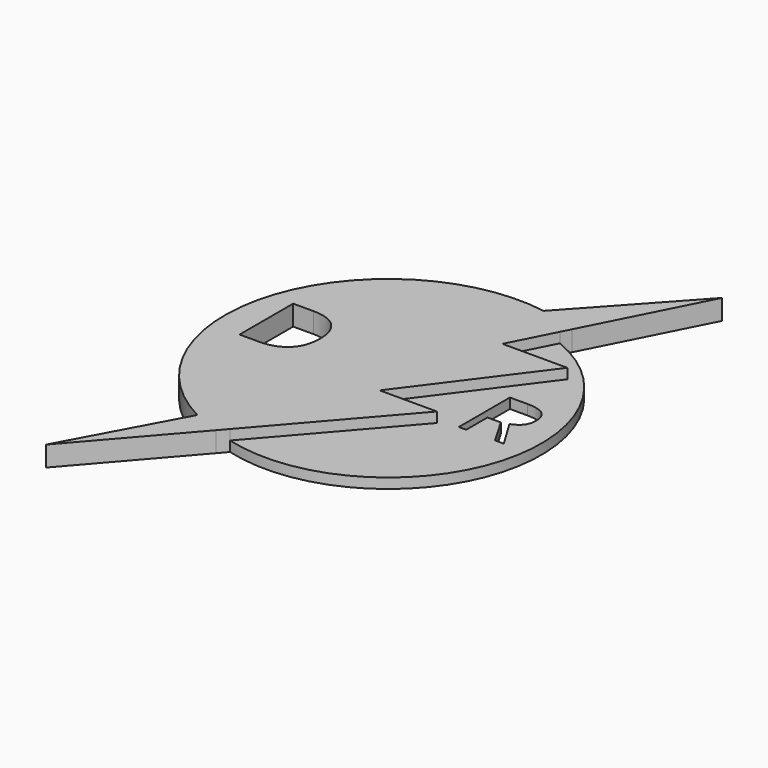
from build123d import *

# Parameters (mm, degrees)
F1_DEPTH = 3.2
F2_DEPTH = 1.6
F3_DEPTH = 2.5


# Not quite as in the source:
# - a feature names something its author has since deleted; it is built from what else it names


with BuildPart() as f1:
    # F0 (on Top) → F1 (new body)
    with BuildSketch(Plane.XY):
        with BuildLine():
            Line((-12.0286401361, 7.7058477327), (2.8731075212, 24.026809333))
            ThreePointArc((2.8731075212, 24.026809333), (-23.1446184854, 7.061795007), (-11.0294978873, -21.5381635686))
            Line((-11.0294978873, -21.5381635686), (-4.3697794008, -9.2094279826))
            Line((-4.3697794008, -9.2094279826), (-18.230907619, -9.2094279826))
            Line((-18.230907619, -9.2094279826), (-2.0674222615, 7.7058477327))
            Line((-2.0674222615, 7.7058477327), (-12.0286401361, 7.7058477327))
        make_face()
        with BuildLine():
            add(Edge.make_bspline(
                [(-14.0679626526, 6.3070743063), (-12.6996164354, 4.9387280892), (-12.6996164354, 2.4824249728)],
                knots=[0, 0, 0, 1, 1, 1], degree=2))
            add(Edge.make_bspline(
                [(-12.6996164354, 2.4824249728), (-12.6996164354, -0.138404107), (-14.1224184292, -1.5252884609)],
                knots=[0, 0, 0, 1, 1, 1], degree=2))
            add(Edge.make_bspline(
                [(-14.1224184292, -1.5252884609), (-15.545220423, -2.9121728148), (-18.2170293788, -2.9121728148)],
                knots=[0, 0, 0, 1, 1, 1], degree=2))
            Line((-18.2170293788, -2.9121728148), (-21.1506895159, -2.9121728148))
            Line((-21.1506895159, -2.9121728148), (-21.1506895159, 7.6754205235))
            Line((-21.1506895159, 7.6754205235), (-17.9065155886, 7.6754205235))
            add(Edge.make_bspline(
                [(-17.9065155886, 7.6754205235), (-15.4363088697, 7.6754205235), (-14.0679626526, 6.3070743063)],
                knots=[0, 0, 0, 1, 1, 1], degree=2))
        make_face(mode=Mode.SUBTRACT)
        with BuildLine():
            ThreePointArc((-11.0294978873, -21.5381635686), (-23.1446184854, 7.061795007), (2.8731075212, 24.026809333))
            Line((2.8731075212, 24.026809333), (4.1858882241, 25.464616759))
            ThreePointArc((4.1858882241, 25.464616759), (-24.5061657926, 8.0880285022), (-11.7940875977, -22.9536024329))
            Line((-11.7940875977, -22.9536024329), (-11.0294978873, -21.5381635686))
        make_face()
        Polygon((4.1858882241, 25.464616759), (2.8731075212, 24.026809333), (-12.0286401361, 7.7058477327), (-2.0674222615, 7.7058477327), (-18.230907619, -9.2094279826), (-4.3697794008, -9.2094279826), (-11.0294978873, -21.5381635686), (-11.7940875977, -22.9536024329), (-21.4260146022, -40.7846085727), (-7.468564605, -24.7020021385), (-6.3056047528, -23.3619704275), (10.7070716166, -3.7589499261), (1.6710584512, -3.7589499261), (15.9755367786, 15.4116954654), (5.7308066454, 15.4116954654), (9.2615315623, 22.3554545173), (9.9925901152, 23.7932030147), (19.2086462315, 41.9181135037), align=None)
    extrude(amount=F1_DEPTH)

    # F0 (on Top) → F2 (join)
    with BuildSketch(Plane.XY):
        with BuildLine():
            ThreePointArc((-6.3056047528, -23.3619704275), (22.9064425811, -7.7998206282), (9.2615315623, 22.3554545173))
            Line((9.2615315623, 22.3554545173), (5.7308066454, 15.4116954654))
            Line((5.7308066454, 15.4116954654), (15.9755367786, 15.4116954654))
            Line((15.9755367786, 15.4116954654), (1.6710584512, -3.7589499261))
            Line((1.6710584512, -3.7589499261), (10.7070716166, -3.7589499261))
            Line((10.7070716166, -3.7589499261), (-6.3056047528, -23.3619704275))
        make_face()
        with BuildLine():
            Line((16.7712777882, 1.29050713), (14.6610901855, 1.29050713))
            Line((14.6610901855, 1.29050713), (14.6610901855, -2.912172582))
            Line((14.6610901855, -2.912172582), (13.4865518028, -2.912172582))
            Line((13.4865518028, -2.912172582), (13.4865518028, 7.1941661569))
            Line((13.4865518028, 7.1941661569), (16.258108476, 7.1941661569))
            add(Edge.make_bspline(
                [(16.258108476, 7.1941661569), (18.1183472327, 7.1941661569), (19.0064398139, 6.4819225426)],
                knots=[0, 0, 0, 1, 1, 1], degree=2))
            add(Edge.make_bspline(
                [(19.0064398139, 6.4819225426), (19.8945323952, 5.7696789282), (19.8945323952, 4.3385558895)],
                knots=[0, 0, 0, 1, 1, 1], degree=2))
            add(Edge.make_bspline(
                [(19.8945323952, 4.3385558895), (19.8945323952, 2.3345412479), (17.8617625766, 1.6289334436)],
                knots=[0, 0, 0, 1, 1, 1], degree=2))
            Line((17.8617625766, 1.6289334436), (20.6067760095, -2.912172582))
            Line((20.6067760095, -2.912172582), (19.2176797679, -2.912172582))
            Line((19.2176797679, -2.912172582), (16.7712777882, 1.29050713))
        make_face(mode=Mode.SUBTRACT)
        with BuildLine():
            Line((-12.0286401361, 7.7058477327), (2.8731075212, 24.026809333))
            ThreePointArc((2.8731075212, 24.026809333), (-23.1446184854, 7.061795007), (-11.0294978873, -21.5381635686))
            Line((-11.0294978873, -21.5381635686), (-4.3697794008, -9.2094279826))
            Line((-4.3697794008, -9.2094279826), (-18.230907619, -9.2094279826))
            Line((-18.230907619, -9.2094279826), (-2.0674222615, 7.7058477327))
            Line((-2.0674222615, 7.7058477327), (-12.0286401361, 7.7058477327))
        make_face()
        with BuildLine():
            add(Edge.make_bspline(
                [(-14.0679626526, 6.3070743063), (-12.6996164354, 4.9387280892), (-12.6996164354, 2.4824249728)],
                knots=[0, 0, 0, 1, 1, 1], degree=2))
            add(Edge.make_bspline(
                [(-12.6996164354, 2.4824249728), (-12.6996164354, -0.138404107), (-14.1224184292, -1.5252884609)],
                knots=[0, 0, 0, 1, 1, 1], degree=2))
            add(Edge.make_bspline(
                [(-14.1224184292, -1.5252884609), (-15.545220423, -2.9121728148), (-18.2170293788, -2.9121728148)],
                knots=[0, 0, 0, 1, 1, 1], degree=2))
            Line((-18.2170293788, -2.9121728148), (-21.1506895159, -2.9121728148))
            Line((-21.1506895159, -2.9121728148), (-21.1506895159, 7.6754205235))
            Line((-21.1506895159, 7.6754205235), (-17.9065155886, 7.6754205235))
            add(Edge.make_bspline(
                [(-17.9065155886, 7.6754205235), (-15.4363088697, 7.6754205235), (-14.0679626526, 6.3070743063)],
                knots=[0, 0, 0, 1, 1, 1], degree=2))
        make_face(mode=Mode.SUBTRACT)
    extrude(amount=F2_DEPTH)

    # F0 (on Top) → F3 (join)
    with BuildSketch(Plane.XY):
        with BuildLine():
            ThreePointArc((-11.0294978873, -21.5381635686), (-23.1446184854, 7.061795007), (2.8731075212, 24.026809333))
            Line((2.8731075212, 24.026809333), (4.1858882241, 25.464616759))
            ThreePointArc((4.1858882241, 25.464616759), (-24.5061657926, 8.0880285022), (-11.7940875977, -22.9536024329))
            Line((-11.7940875977, -22.9536024329), (-11.0294978873, -21.5381635686))
        make_face()
    extrude(amount=F3_DEPTH)


solid = f1.part
